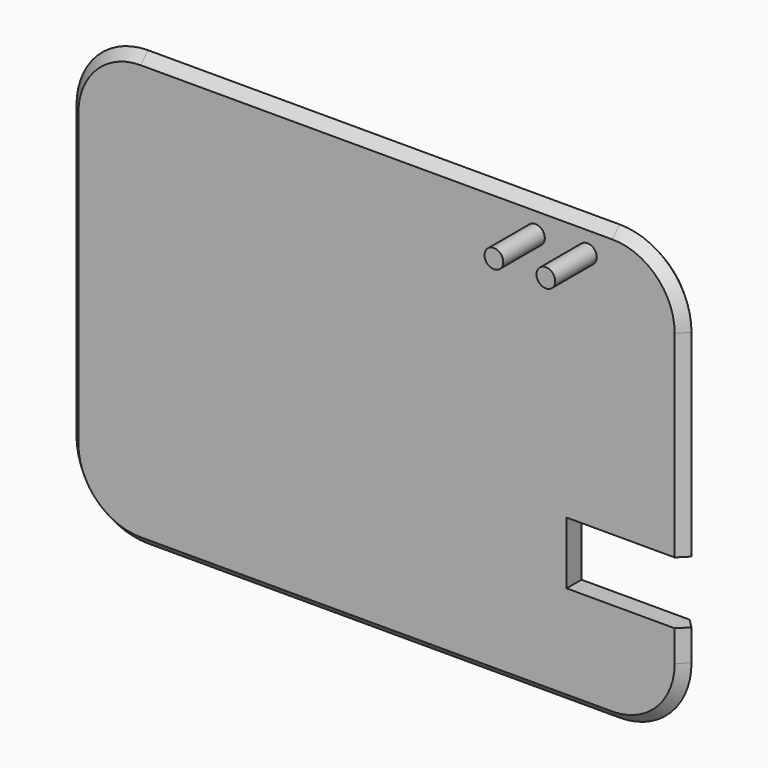
from build123d import *

# Parameters (mm, degrees)
F1_DEPTH     = 9
F2_R         = 4.5
F3_DEPTH     = 25
F4_W         = 57
F4_H         = 30
F5_DEPTH     = 25
F6_SIZE      = 5
F7_T1_DEPTH  = 227
F7_T3_DEPTH  = 107.8584149398
F7_T5_DEPTH  = 27.8584149398
F7_T7_DEPTH  = 140
F7_T10_ANGLE = 90
F7_T12_ANGLE = 90
F7_T14_ANGLE = 90
F7_T16_ANGLE = 90


# Not quite as in the source:
# - a fillet or chamfer that OpenCascade refuses, or shapes differently, is made with other operations: its cross-section is extruded or revolved along the edge and cut away or added


with BuildPart() as f1:
    # F0 (on Front) → F1 (new body)
    with BuildSketch(Plane.XZ):
        with BuildLine():
            Line((113.7409908921, 84.5945477496), (-113.2590091079, 84.5945477496))
            ThreePointArc((-113.2590091079, 84.5945477496), (-138.0077464495, 74.3432850912), (-148.2590091079, 49.5945477496))
            Line((-148.2590091079, 49.5945477496), (-148.2590091079, -90.4054522504))
            ThreePointArc((-148.2590091079, -90.4054522504), (-138.0077464495, -115.1541895919), (-113.2590091079, -125.4054522504))
            Line((-113.2590091079, -125.4054522504), (113.7409908921, -125.4054522504))
            ThreePointArc((113.7409908921, -125.4054522504), (138.4897282336, -115.1541895919), (148.7409908921, -90.4054522504))
            Line((148.7409908921, -90.4054522504), (148.7409908921, 49.5945477496))
            ThreePointArc((148.7409908921, 49.5945477496), (138.4897282336, 74.3432850912), (113.7409908921, 84.5945477496))
        make_face()
    extrude(amount=F1_DEPTH)

    # F2 (on face) → F3 (join)
    with BuildSketch(Plane.XZ.offset(9)):
        with Locations((101.7409908921, 69.5945477496)):
            Circle(F2_R)
        with Locations((76.7409908921, 69.5945477496)):
            Circle(F2_R)
    extrude(amount=F3_DEPTH)

    # F4 (on face) → F5 (cut)
    with BuildSketch(Plane.XZ.offset(9)):
        with Locations((120.2409908921, -60.4054522504)):
            Rectangle(F4_W, F4_H)
    extrude(amount=-F5_DEPTH, mode=Mode.SUBTRACT)

    # F6
    f6_edges = [f1.edges().sort_by_distance(p)[0] for p in [
        (0.240991, -9, 84.594548),
    ]]
    chamfer(f6_edges, length=F6_SIZE)

    # F7: chamfer of 5 on 9 edges, made by hand

    # F7_s2 → F7_t1 (cut)
    with BuildSketch(Plane.YZ.offset(-113.2590091079)):
        with BuildLine():
            Line((-5.1414213562, 84.7359691059), (0.1414213562, 79.4531263934))
            Line((0.1414213562, 79.4531263934), (0.2414213562, 79.4531263934))
            ThreePointArc((0.2414213562, 79.4531263934), (0.1, 82.0238370715), (0.1, 84.5945477496))
            Line((0.1, 84.5945477496), (0, 84.6945477496))
            ThreePointArc((0, 84.6945477496), (-2.5707106781, 84.6945477496), (-5.1414213562, 84.8359691059))
            Line((-5.1414213562, 84.8359691059), (-5.1414213562, 84.7359691059))
        make_face()
        with BuildLine():
            Line((0.1414213562, -120.2640308941), (-5.1414213562, -125.5468736066))
            Line((-5.1414213562, -125.5468736066), (-5.1414213562, -125.6468736066))
            ThreePointArc((-5.1414213562, -125.6468736066), (-2.5707106781, -125.5054522504), (0, -125.5054522504))
            Line((0, -125.5054522504), (0.1, -125.4054522504))
            ThreePointArc((0.1, -125.4054522504), (0.1, -122.8347415723), (0.2414213562, -120.2640308941))
            Line((0.2414213562, -120.2640308941), (0.1414213562, -120.2640308941))
        make_face()
    extrude(amount=F7_T1_DEPTH, mode=Mode.SUBTRACT)

    # F7_s4 → F7_t3 (cut)
    with BuildSketch(Plane.XY.offset(-58.2638671902)):
        with BuildLine():
            Line((143.5995695358, 0.1414213562), (148.8824122483, -5.1414213562))
            Line((148.8824122483, -5.1414213562), (148.9824122483, -5.1414213562))
            ThreePointArc((148.9824122483, -5.1414213562), (148.8409908921, -2.5707106781), (148.8409908921, 0))
            Line((148.8409908921, 0), (148.7409908921, 0.1))
            ThreePointArc((148.7409908921, 0.1), (146.1702802139, 0.1), (143.5995695358, 0.2414213562))
            Line((143.5995695358, 0.2414213562), (143.5995695358, 0.1414213562))
        make_face()
    extrude(amount=F7_T3_DEPTH, mode=Mode.SUBTRACT)

    # F7_s6 → F7_t5 (cut)
    with BuildSketch(Plane.XY.offset(-90.4054522504)):
        with BuildLine():
            Line((143.5995695358, 0.1414213562), (148.8824122483, -5.1414213562))
            Line((148.8824122483, -5.1414213562), (148.9824122483, -5.1414213562))
            ThreePointArc((148.9824122483, -5.1414213562), (148.8409908921, -2.5707106781), (148.8409908921, 0))
            Line((148.8409908921, 0), (148.7409908921, 0.1))
            ThreePointArc((148.7409908921, 0.1), (146.1702802139, 0.1), (143.5995695358, 0.2414213562))
            Line((143.5995695358, 0.2414213562), (143.5995695358, 0.1414213562))
        make_face()
    extrude(amount=F7_T5_DEPTH, mode=Mode.SUBTRACT)

    # F7_s8 → F7_t7 (cut)
    with BuildSketch(Plane.XY.offset(-90.4054522504)):
        with BuildLine():
            Line((-143.1175877517, 0.1414213562), (-148.4004304642, -5.1414213562))
            Line((-148.4004304642, -5.1414213562), (-148.5004304642, -5.1414213562))
            ThreePointArc((-148.5004304642, -5.1414213562), (-148.3590091079, -2.5707106781), (-148.3590091079, 0))
            Line((-148.3590091079, 0), (-148.2590091079, 0.1))
            ThreePointArc((-148.2590091079, 0.1), (-145.6882984298, 0.1), (-143.1175877517, 0.2414213562))
            Line((-143.1175877517, 0.2414213562), (-143.1175877517, 0.1414213562))
        make_face()
    extrude(amount=F7_T7_DEPTH, mode=Mode.SUBTRACT)

    # F7_s9 → F7_t10 (revolve, cut)
    with BuildSketch(Plane.XY.offset(49.5945477496)):
        with BuildLine():
            Line((148.8824122483, -5.1414213562), (143.5995695358, 0.1414213562))
            Line((143.5995695358, 0.1414213562), (143.5995695358, 0.2414213562))
            ThreePointArc((143.5995695358, 0.2414213562), (146.1702802139, 0.1), (148.7409908921, 0.1))
            Line((148.7409908921, 0.1), (148.8409908921, 0))
            ThreePointArc((148.8409908921, 0), (148.8409908921, -2.5707106781), (148.9824122483, -5.1414213562))
            Line((148.9824122483, -5.1414213562), (148.8824122483, -5.1414213562))
        make_face()
    revolve(axis=Axis((113.7409908921, 0, 49.5945477496), (0, -1, 0)), revolution_arc=F7_T10_ANGLE, mode=Mode.SUBTRACT)

    # F7_s11 → F7_t12 (revolve, cut)
    with BuildSketch(Plane.YZ.offset(113.7409908921)):
        with BuildLine():
            Line((0.1414213562, -120.2640308941), (-5.1414213562, -125.5468736066))
            Line((-5.1414213562, -125.5468736066), (-5.1414213562, -125.6468736066))
            ThreePointArc((-5.1414213562, -125.6468736066), (-2.5707106781, -125.5054522504), (0, -125.5054522504))
            Line((0, -125.5054522504), (0.1, -125.4054522504))
            ThreePointArc((0.1, -125.4054522504), (0.1, -122.8347415723), (0.2414213562, -120.2640308941))
            Line((0.2414213562, -120.2640308941), (0.1414213562, -120.2640308941))
        make_face()
    revolve(axis=Axis((113.7409908921, 0, -90.4054522504), (0, -1, 0)), revolution_arc=F7_T12_ANGLE, mode=Mode.SUBTRACT)

    # F7_s13 → F7_t14 (revolve, cut)
    with BuildSketch(Plane.XY.offset(-90.4054522504)):
        with BuildLine():
            Line((-143.1175877517, 0.1414213562), (-148.4004304642, -5.1414213562))
            Line((-148.4004304642, -5.1414213562), (-148.5004304642, -5.1414213562))
            ThreePointArc((-148.5004304642, -5.1414213562), (-148.3590091079, -2.5707106781), (-148.3590091079, 0))
            Line((-148.3590091079, 0), (-148.2590091079, 0.1))
            ThreePointArc((-148.2590091079, 0.1), (-145.6882984298, 0.1), (-143.1175877517, 0.2414213562))
            Line((-143.1175877517, 0.2414213562), (-143.1175877517, 0.1414213562))
        make_face()
    revolve(axis=Axis((-113.2590091079, 0, -90.4054522504), (0, -1, 0)), revolution_arc=F7_T14_ANGLE, mode=Mode.SUBTRACT)

    # F7_s15 → F7_t16 (revolve, cut)
    with BuildSketch(Plane.YZ.offset(-113.2590091079)):
        with BuildLine():
            Line((0.1414213562, 79.4531263934), (-5.1414213562, 84.7359691059))
            Line((-5.1414213562, 84.7359691059), (-5.1414213562, 84.8359691059))
            ThreePointArc((-5.1414213562, 84.8359691059), (-2.5707106781, 84.6945477496), (0, 84.6945477496))
            Line((0, 84.6945477496), (0.1, 84.5945477496))
            ThreePointArc((0.1, 84.5945477496), (0.1, 82.0238370715), (0.2414213562, 79.4531263934))
            Line((0.2414213562, 79.4531263934), (0.1414213562, 79.4531263934))
        make_face()
    revolve(axis=Axis((-113.2590091079, 0, 49.5945477496), (0, -1, 0)), revolution_arc=F7_T16_ANGLE, mode=Mode.SUBTRACT)


solid = f1.part
